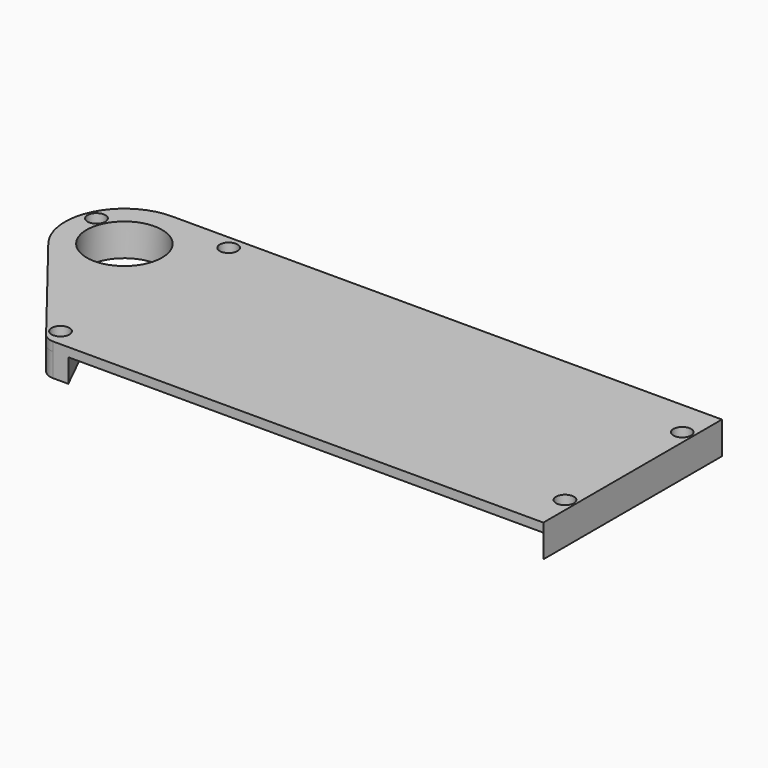
from build123d import *

# Parameters (mm, degrees)
F0_R           = 12.7
F1_DEPTH       = 7.9
F1_FACE_R      = 12.7
F2_DEPTH       = 3
F3_DEPTH       = 3
F4_R           = 5
F8_D           = 3.3
F8_CBORE_D     = 6
F8_CBORE_DEPTH = 3.3


# Not quite as in the source:
# - a feature names something its author has since deleted; it is built from what else it names


with BuildPart() as f1:
    # F0 (on Top) → F1 (new body)
    with BuildSketch(Plane.XY):
        with BuildLine():
            ThreePointArc((-82.519158721, -19.8666825891), (-82.3199649398, 11.4193737584), (-65.6162592679, 37.8739237785))
            Line((-65.6162592679, 37.8739237785), (-99.2088739193, 37.8739237785))
            ThreePointArc((-99.2088739193, 37.8739237785), (-117.1879721114, 26.6373104948), (-114.9666717313, 5.5523567478))
            Line((-114.9666717313, 5.5523567478), (-81.4747432756, -37.2867286205))
            Line((-81.4747432756, -37.2867286205), (-73.9695476283, -37.2867286205))
            Line((-73.9695476283, -37.2867286205), (-82.519158721, -19.8666825891))
        make_face()
        with Locations((-99.2088739193, 17.8719250206)):
            Circle(F0_R, mode=Mode.SUBTRACT)
    extrude(amount=-F1_DEPTH)



with BuildPart() as f1b:
    # F0 (on Top) → F1, piece 2 (new body)
    with BuildSketch(Plane.XY):
        with BuildLine():
            Line((86, -37.2867286205), (86, 37.8739237785))
            ThreePointArc((86, 37.8739237785), (76.5230858808, 21.4851908555), (70.8448413014, 3.4252903424))
            ThreePointArc((70.8448413014, 3.4252903424), (70.5487291916, -0.5692843065), (71.2877699379, -4.5060504646))
            ThreePointArc((71.2877699379, -4.5060504646), (77.4631412951, -21.4263167299), (86, -37.2867286205))
        make_face()
    extrude(amount=-F1_DEPTH)


with BuildPart() as f1_1:
    add(f1.part)

    add(f1b.part)  # F2 merges F1b
    # F0 (on Top) + F1_face (on face) → F2 (join)
    with BuildSketch(Plane.XY):
        with BuildLine():
            ThreePointArc((70.8448413014, 3.4252903424), (76.5230858808, 21.4851908555), (86, 37.8739237785))
            Line((86, 37.8739237785), (-65.6162592679, 37.8739237785))
            ThreePointArc((-65.6162592679, 37.8739237785), (-82.3199649398, 11.4193737584), (-82.519158721, -19.8666825891))
            Line((-82.519158721, -19.8666825891), (-73.9695476283, -37.2867286205))
            Line((-73.9695476283, -37.2867286205), (86, -37.2867286205))
            ThreePointArc((86, -37.2867286205), (77.4631412951, -21.4263167299), (71.2877699379, -4.5060504646))
            ThreePointArc((71.2877699379, -4.5060504646), (70.5487291916, -0.5692843065), (70.8448413014, 3.4252903424))
        make_face()
    with BuildSketch(Plane(origin=(-93.510683798, 7.7887517246, 0), x_dir=(1, 0, 0), z_dir=(0, 0, 1))):
        with BuildLine():
            ThreePointArc((10.9915250771, -27.6554343137), (11.1907188583, 3.6306220338), (27.8944245301, 30.0851720539))
            Line((27.8944245301, 30.0851720539), (-5.6981901212, 30.0851720539))
            ThreePointArc((-5.6981901212, 30.0851720539), (-23.6772883134, 18.8485587701), (-21.4559879333, -2.2363949769))
            Line((-21.4559879333, -2.2363949769), (12.0359405224, -45.0754803451))
            Line((12.0359405224, -45.0754803451), (19.5411361698, -45.0754803451))
            Line((19.5411361698, -45.0754803451), (10.9915250771, -27.6554343137))
        make_face()
        with Locations((-5.6981901212, 10.083173296)):
            Circle(F1_FACE_R, mode=Mode.SUBTRACT)
    extrude(amount=F2_DEPTH)

    # F4
    f4_edges = [f1_1.edges().sort_by_distance(p)[0] for p in [
        (-81.474743, -37.286729, -2.45),
    ]]
    fillet(f4_edges, radius=F4_R)


with BuildPart() as f3:
    # F0 (on Top) → F3 (new body)
    with BuildSketch(Plane.XY):
        with BuildLine():
            Line((86, -37.2867286205), (86, 37.8739237785))
            ThreePointArc((86, 37.8739237785), (76.5230858808, 21.4851908555), (70.8448413014, 3.4252903424))
            ThreePointArc((70.8448413014, 3.4252903424), (70.5487291916, -0.5692843065), (71.2877699379, -4.5060504646))
            ThreePointArc((71.2877699379, -4.5060504646), (77.4631412951, -21.4263167299), (86, -37.2867286205))
        make_face()
    extrude(amount=F3_DEPTH)


with BuildPart() as f1_2:
    add(f1_1.part)

    # F6: union F3
    add(f3.part)

    # F8 (through all)
    with Locations(Plane.XY.offset(3)):
        with Locations((-76.3588739193, 33.2139237785), (-113.9428039086, 24.5539237785), (-81.1954878403, -31.5067286205), (82.39, -23.6667286205), (82.39, 25.7039237785)):
            CounterBoreHole(F8_D / 2, F8_CBORE_D / 2, F8_CBORE_DEPTH)


solid = f1_2.part
